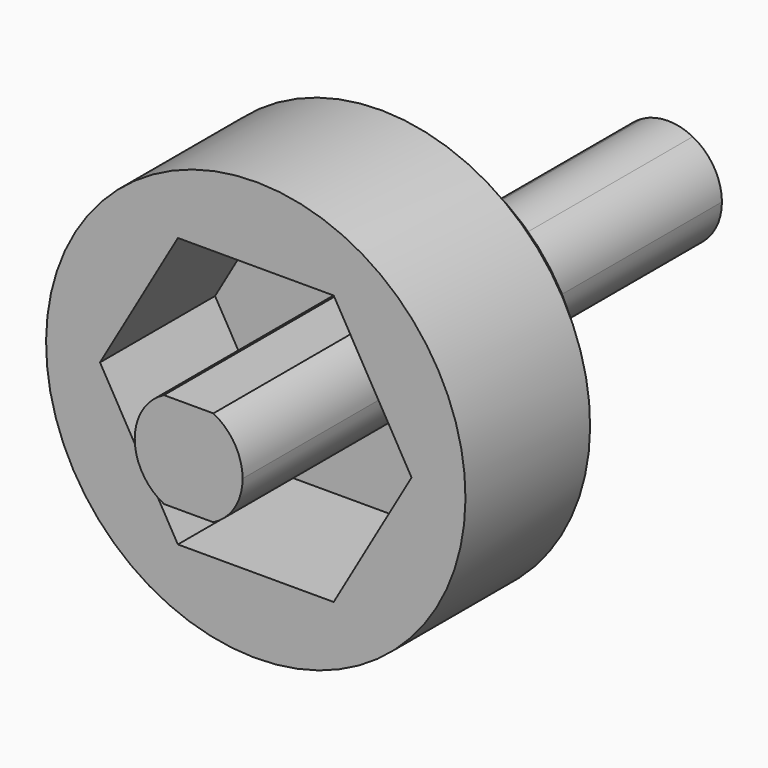
from build123d import *

# Parameters (mm, degrees)
F1_DEPTH      = 16
F2_DEPTH      = 12
F3_SIZE       = 3
F4_DEPTH      = 7
F4_DEPTH_BACK = 22
F5_START      = -22
F5_DEPTH      = 21
F6_W          = 1
F6_H          = 0.5


# Not quite as in the source:
# - a feature names something its author has since deleted; it is built from what else it names


with BuildPart() as f1:
    # F0 (on Front) → F1 (new body)
    with BuildSketch(Plane.XZ):
        with BuildLine():
            ThreePointArc((1.668909711, 17.4202393892), (-8.75, 15.1554445662), (-15.9208247065, 7.2648014882))
            ThreePointArc((-15.9208247065, 7.2648014882), (8.75, -15.1554445662), (1.668909711, 17.4202393892))
        make_face()
        Polygon((-13, 0), (-6.5, 11.2583302492), (6.5, 11.2583302492), (13, 0), (6.5, -11.2583302492), (-6.5, -11.2583302492), align=None, mode=Mode.SUBTRACT)
        Polygon((6.5, 11.2583302492), (-6.5, 11.2583302492), (-13, 0), (-6.5, -11.2583302492), (6.5, -11.2583302492), (13, 0), align=None)
        with BuildLine():
            ThreePointArc((-2.0615528128, -4), (-4.5, 0), (-2.0615528128, 4))
            ThreePointArc((-2.0615528128, 4), (0, 4.5), (2.0615528128, 4))
            ThreePointArc((2.0615528128, 4), (3.8423292192, 2.3423292192), (4.5, 0))
            ThreePointArc((4.5, 0), (3.8423292192, -2.3423292192), (2.0615528128, -4))
            ThreePointArc((2.0615528128, -4), (0, -4.5), (-2.0615528128, -4))
        make_face(mode=Mode.SUBTRACT)
        with BuildLine():
            ThreePointArc((2.0615528128, 4), (0, 4.5), (-2.0615528128, 4))
            Line((-2.0615528128, 4), (2.0615528128, 4))
        make_face()
        with BuildLine():
            Line((2.0615528128, -4), (-2.0615528128, -4))
            ThreePointArc((-2.0615528128, -4), (0, -4.5), (2.0615528128, -4))
        make_face()
    extrude(amount=-F1_DEPTH)

    # F0 (on Front) → F2 (cut)
    with BuildSketch(Plane.XZ):
        Polygon((6.5, 11.2583302492), (-6.5, 11.2583302492), (-13, 0), (-6.5, -11.2583302492), (6.5, -11.2583302492), (13, 0), align=None)
        with BuildLine():
            ThreePointArc((-2.0615528128, -4), (-4.5, 0), (-2.0615528128, 4))
            ThreePointArc((-2.0615528128, 4), (0, 4.5), (2.0615528128, 4))
            ThreePointArc((2.0615528128, 4), (3.8423292192, 2.3423292192), (4.5, 0))
            ThreePointArc((4.5, 0), (3.8423292192, -2.3423292192), (2.0615528128, -4))
            ThreePointArc((2.0615528128, -4), (0, -4.5), (-2.0615528128, -4))
        make_face(mode=Mode.SUBTRACT)
        with BuildLine():
            ThreePointArc((2.0615528128, 4), (0, 4.5), (-2.0615528128, 4))
            Line((-2.0615528128, 4), (2.0615528128, 4))
        make_face()
        with BuildLine():
            Line((2.0615528128, -4), (-2.0615528128, -4))
            ThreePointArc((-2.0615528128, -4), (0, -4.5), (2.0615528128, -4))
        make_face()
    extrude(amount=-F2_DEPTH, mode=Mode.SUBTRACT)

    # F3
    f3_edges = [f1.edges().sort_by_distance(p)[0] for p in [
        (-1.66891, 16, -17.420239),
    ]]
    chamfer(f3_edges, length=F3_SIZE)


with BuildPart() as f4:
    # F0 (on Front) → F4 (new body, two sides)
    with BuildSketch(Plane.XZ) as f4_sk:
        with BuildLine():
            Line((2.0615528128, 4), (-2.0615528128, 4))
            ThreePointArc((-2.0615528128, 4), (-4.5, 0), (-2.0615528128, -4))
            Line((-2.0615528128, -4), (2.0615528128, -4))
            ThreePointArc((2.0615528128, -4), (3.8423292192, -2.3423292192), (4.5, 0))
            ThreePointArc((4.5, 0), (3.8423292192, 2.3423292192), (2.0615528128, 4))
        make_face()
    extrude(amount=F4_DEPTH)
    extrude(f4_sk.sketch, amount=-F4_DEPTH_BACK)

    # F0 (on Front) → F5 (join)
    with BuildSketch(Plane.XZ.offset(F5_START)):
        with BuildLine():
            Line((2.0615528128, 4), (-2.0615528128, 4))
            ThreePointArc((-2.0615528128, 4), (-4.5, 0), (-2.0615528128, -4))
            Line((-2.0615528128, -4), (2.0615528128, -4))
            ThreePointArc((2.0615528128, -4), (3.8423292192, -2.3423292192), (4.5, 0))
            ThreePointArc((4.5, 0), (3.8423292192, 2.3423292192), (2.0615528128, 4))
        make_face()
        with BuildLine():
            ThreePointArc((2.0615528128, 4), (0, 4.5), (-2.0615528128, 4))
            Line((-2.0615528128, 4), (2.0615528128, 4))
        make_face()
    extrude(amount=-F5_DEPTH)

    # F6 (on Right) → F7 (revolve, cut)
    with BuildSketch(Plane.YZ):
        with Locations((11.5, -2.75)):
            Rectangle(F6_W, F6_H)
        with Locations((20.5, -2.75)):
            Rectangle(F6_W, F6_H)
        with Locations((25.5, -2.75)):
            Rectangle(F6_W, F6_H)
        with Locations((27.5, -2.75)):
            Rectangle(F6_W, F6_H)
        with Locations((34.5, -2.75)):
            Rectangle(F6_W, F6_H)
        with Locations((39.5, -2.75)):
            Rectangle(F6_W, F6_H)
        Polygon((43, -3), (43, -2.5), (42.5, -3), align=None)
    revolve(axis=Axis((0, 43, 0), (0, -1, 0)), mode=Mode.SUBTRACT)


solid = Compound([f1.part, f4.part])
